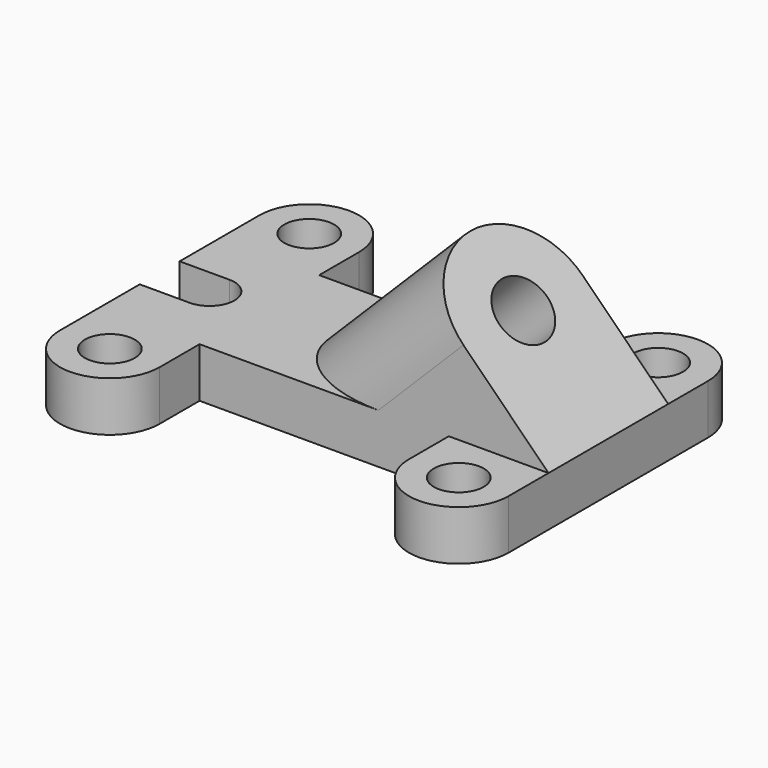
from build123d import *

# Parameters (mm, degrees)
F0_R     = 0.25
F1_DEPTH = 0.5
F3_DEPTH = 2
F4_W     = 4.4533928877
F4_H     = 2.379073936
F5_DEPTH = 0.5
F7_REACH = 4.5971940777
F8_R     = 0.3
F9_DEPTH = 25


with BuildPart() as f1:
    # F0 (on Top) → F1 (new body)
    with BuildSketch(Plane.XY):
        with BuildLine():
            Line((-0.5, 1), (-0.5, 0))
            ThreePointArc((-0.5, 0), (0, -0.5), (0.5, 0))
            Line((0.5, 0), (0.5, 0.5))
            Line((0.5, 0.5), (3, 0.5))
            Line((3, 0.5), (3, 0))
            ThreePointArc((3, 0), (3.5, -0.5), (4, 0))
            Line((4, 0), (4, 2.5))
            ThreePointArc((4, 2.5), (3.5, 3), (3, 2.5))
            Line((3, 2.5), (3, 2))
            Line((3, 2), (0.5, 2))
            Line((0.5, 2), (0.5, 2.5))
            ThreePointArc((0.5, 2.5), (0, 3), (-0.5, 2.5))
            Line((-0.5, 2.5), (-0.5, 1.5))
            Line((-0.5, 1.5), (0, 1.5))
            ThreePointArc((0, 1.5), (0.25, 1.25), (0, 1))
            Line((0, 1), (-0.5, 1))
        make_face()
        Circle(F0_R, mode=Mode.SUBTRACT)
        with Locations((3.5, 0)):
            Circle(F0_R, mode=Mode.SUBTRACT)
        with Locations((0, 2.5)):
            Circle(F0_R, mode=Mode.SUBTRACT)
        with Locations((3.5, 2.5)):
            Circle(F0_R, mode=Mode.SUBTRACT)
    extrude(amount=F1_DEPTH)

    # F2 (on Front) → F3 (join)
    with BuildSketch(Plane.XZ):
        Polygon((2.6167841171, 1.8832158829), (1.2335682341, 0.5), (4, 0.5), align=None)
    extrude(amount=-F3_DEPTH)

    # F4 (on Front) → F5 (cut)
    with BuildSketch(Plane.XZ):
        with Locations((1.7733035561, 1.689536968)):
            Rectangle(F4_W, F4_H)
    extrude(amount=-F5_DEPTH, mode=Mode.SUBTRACT)

    f7_end = Plane(origin=(0.2759630483, 1.25, 0.5), x_dir=(1, 0, 0), z_dir=(0, 0, 1))
    # F6 (on face) → F7 (cut, up to a plane its end follows)
    with BuildSketch(Plane(origin=(2.25, 0, 2.25), x_dir=(0.7071067812, 0, -0.7071067812), z_dir=(0.7071067812, 0, 0.7071067812))):
        with BuildLine():
            ThreePointArc((1.2687110728, 0.5), (0.7383809869, 0.7196699141), (0.5187110728, 1.25))
            Line((0.5187110728, 1.25), (0.5187110728, 0.5))
            Line((0.5187110728, 0.5), (1.2687110728, 0.5))
        make_face()
        with BuildLine():
            ThreePointArc((0.5187110728, 1.25), (0.7383809869, 1.7803300859), (1.2687110728, 2))
            Line((1.2687110728, 2), (0.5187110728, 2))
            Line((0.5187110728, 2), (0.5187110728, 1.25))
        make_face()
    f7_long = extrude(amount=-F7_REACH, mode=Mode.PRIVATE)
    add(split(f7_long, bisect_by=f7_end, keep=Keep.TOP, mode=Mode.PRIVATE), mode=Mode.SUBTRACT)

    # F8 (on face) → F9 (cut)
    with BuildSketch(Plane(origin=(2.25, 0, 2.25), x_dir=(0.7071067812, 0, -0.7071067812), z_dir=(0.7071067812, 0, 0.7071067812))):
        with Locations((1.2687110728, 1.25)):
            Circle(F8_R)
    extrude(amount=-F9_DEPTH, mode=Mode.SUBTRACT)


solid = f1.part
